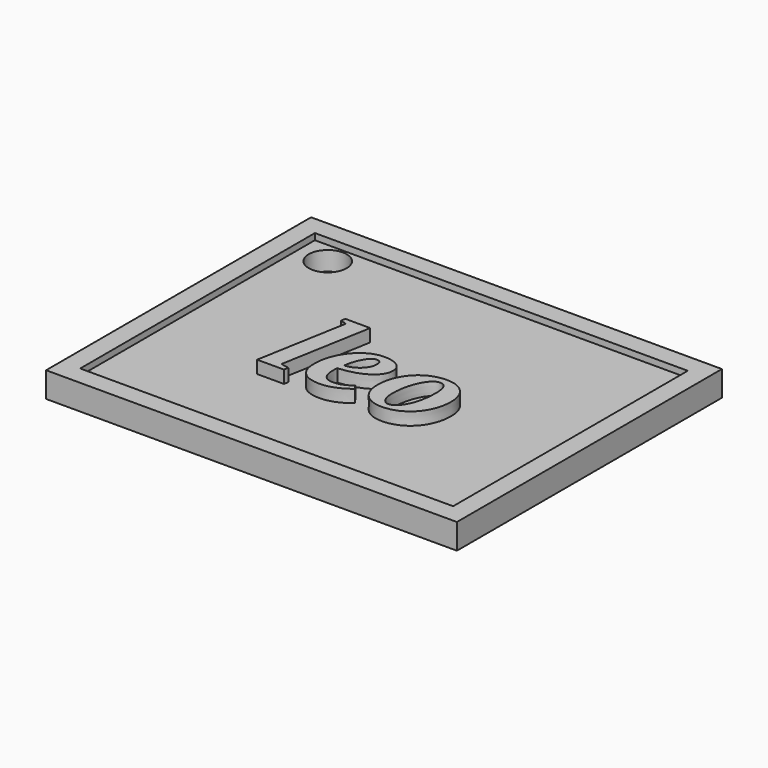
from build123d import *

# Parameters (mm, degrees)
F0_W         = 64.9619624019
F0_H         = 52.3797534406
F1_DEPTH     = 4
F2_T         = -3
F3_TEXT_SIZE = 22.0905187436
F4_DEPTH     = 2
F6_D         = 6


# Not quite as in the source:
# - Text() gives the source's letters only with a copy of the font that has no kerning and outlines rounded to 1/6400 em; it was checked with that copy


with BuildPart() as f1:
    # F0 (on Top) → F1 (new body)
    with BuildSketch(Plane.XY):
        with Locations((32.4809812009, -26.1898767203)):
            Rectangle(F0_W, F0_H)
    extrude(amount=F1_DEPTH)

    # F2
    f2_openings = [f1.faces().sort_by_distance(p)[0] for p in [
        (32.480981, -26.189877, 4),
    ]]
    offset(amount=F2_T, openings=f2_openings)

    # F3 (on face) → F4 (join)
    with BuildSketch(Plane.XY.offset(3)):
        with Locations((19.2995676771, -35.3987086564)):
            Text('leo', F3_TEXT_SIZE, font='Tinos', font_style=FontStyle.BOLDITALIC, text_align=(TextAlign.LEFT, TextAlign.BOTTOM))
    extrude(amount=F4_DEPTH)

    # F6 (through all)
    with Locations(Plane.XY.offset(3)):
        with Locations((7.7438922599, -6.3931019977)):
            Hole(F6_D / 2)


solid = f1.part
